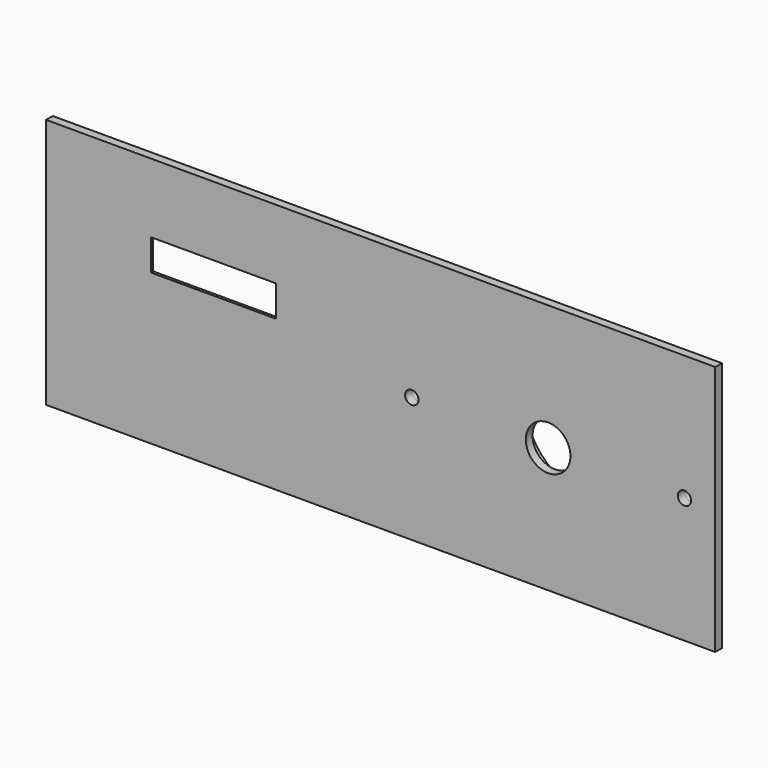
from build123d import *

# Parameters (mm, degrees)
F0_W      = 120
F0_H      = 1.5
F1_DEPTH  = 45
F2_R      = 4
F3_DEPTH  = 25
F4_R      = 1.2
F5_DEPTH  = 25
F6_W      = 11.7
F6_H      = 6.5
F6_R      = 1.2
F7_DEPTH  = 1.6
F8_DEPTH  = 5.9
F9_W      = 32
F9_H      = 28.2
F10_DEPTH = 1.6
F11_R     = 11.25
F12_DEPTH = 25
F13_R     = 1.1
F14_DEPTH = 25
F15_W     = 22.384
F15_H     = 5.584
F16_DEPTH = 25
F17_W     = 30
F17_H     = 11.5
F17_W_2   = 22.384
F17_H_2   = 5.584
F18_DEPTH = 1


with BuildPart() as f1:
    # F0 (on Top) → F1 (new body)
    with BuildSketch(Plane.XY):
        Rectangle(F0_W, F0_H)
    extrude(amount=F1_DEPTH)

    # F2 (on face) → F3 (cut)
    with BuildSketch(Plane.XZ.offset(0.75)):
        with Locations((30.0324354321, 22.5)):
            Circle(F2_R)
    extrude(amount=-F3_DEPTH, mode=Mode.SUBTRACT)

    # F4 (on face) → F5 (cut)
    with BuildSketch(Plane.XZ.offset(0.75)):
        with Locations((5.5824354321, 22.5)):
            Circle(F4_R)
        with Locations((54.4824354321, 22.5)):
            Circle(F4_R)
    extrude(amount=-F5_DEPTH, mode=Mode.SUBTRACT)

    # F15 (on face) → F16 (cut)
    with BuildSketch(Plane.XZ.offset(0.75)):
        with Locations((-30, 29.792)):
            Rectangle(F15_W, F15_H)
    extrude(amount=-F16_DEPTH, mode=Mode.SUBTRACT)

    # F17 (on face) → F18 (cut)
    with BuildSketch(Plane(origin=(0, 0.75, 0), x_dir=(-1, 0, 0), z_dir=(0, 1, 0))):
        with Locations((28.192, 28.834)):
            Rectangle(F17_W, F17_H)
        with Locations((30, 29.792)):
            Rectangle(F17_W_2, F17_H_2, mode=Mode.SUBTRACT)
    extrude(amount=-F18_DEPTH, mode=Mode.SUBTRACT)


with BuildPart() as f7:
    # F6 (on face) → F7 (new body)
    with BuildSketch(Plane(origin=(0, 0.75, 0), x_dir=(-1, 0, 0), z_dir=(0, 1, 0))):
        with Locations((-51.8824354321, 22.5)):
            Rectangle(F6_W, F6_H)
        with Locations((-54.4824354321, 22.5)):
            Circle(F6_R, mode=Mode.SUBTRACT)
    extrude(amount=F7_DEPTH)

    # F6 (on face) → F8 (join)
    with BuildSketch(Plane(origin=(0, 0.75, 0), x_dir=(-1, 0, 0), z_dir=(0, 1, 0))):
        Polygon((-46.0324354321, 36.6), (-46.0324354321, 25.75), (-46.0324354321, 19.25), (-46.0324354321, 8.4), (-44.4324354321, 8.4), (-44.4324354321, 36.6), align=None)
    extrude(amount=F8_DEPTH)



with BuildPart() as f7b:
    # F6 (on face) → F7, piece 2 (new body)
    with BuildSketch(Plane(origin=(0, 0.75, 0), x_dir=(-1, 0, 0), z_dir=(0, 1, 0))):
        with Locations((-8.1824354321, 22.5)):
            Rectangle(F6_W, F6_H)
        with Locations((-5.5824354321, 22.5)):
            Circle(F6_R, mode=Mode.SUBTRACT)
    extrude(amount=F7_DEPTH)

    # F6 (on face) → F8, piece 2 (join)
    with BuildSketch(Plane(origin=(0, 0.75, 0), x_dir=(-1, 0, 0), z_dir=(0, 1, 0))):
        Polygon((-14.0324354321, 25.75), (-14.0324354321, 36.6), (-15.6324354321, 36.6), (-15.6324354321, 8.4), (-14.0324354321, 8.4), (-14.0324354321, 19.25), align=None)
    extrude(amount=F8_DEPTH)


with BuildPart() as f7_1:
    add(f7.part)

    add(f7b.part)  # F10 merges F7b
    # F9 (on face) → F10 (join)
    with BuildSketch(Plane(origin=(0, 6.65, 0), x_dir=(-1, 0, 0), z_dir=(0, 1, 0))):
        with Locations((-30.0324354321, 22.5)):
            Rectangle(F9_W, F9_H)
    extrude(amount=F10_DEPTH)

    # F11 (on face) → F12 (cut)
    with BuildSketch(Plane(origin=(0, 8.25, 0), x_dir=(-1, 0, 0), z_dir=(0, 1, 0))):
        with Locations((-30.0324354321, 22.5)):
            Circle(F11_R)
    extrude(amount=-F12_DEPTH, mode=Mode.SUBTRACT)

    # F13 (on face) → F14 (cut)
    with BuildSketch(Plane(origin=(0, 8.25, 0), x_dir=(-1, 0, 0), z_dir=(0, 1, 0))):
        with Locations((-41.5324354321, 34)):
            Circle(F13_R)
        with Locations((-18.5324354321, 34)):
            Circle(F13_R)
        with Locations((-18.5324354321, 11)):
            Circle(F13_R)
        with Locations((-41.5324354321, 11)):
            Circle(F13_R)
    extrude(amount=-F14_DEPTH, mode=Mode.SUBTRACT)


solid = Compound([f1.part, f7_1.part])
